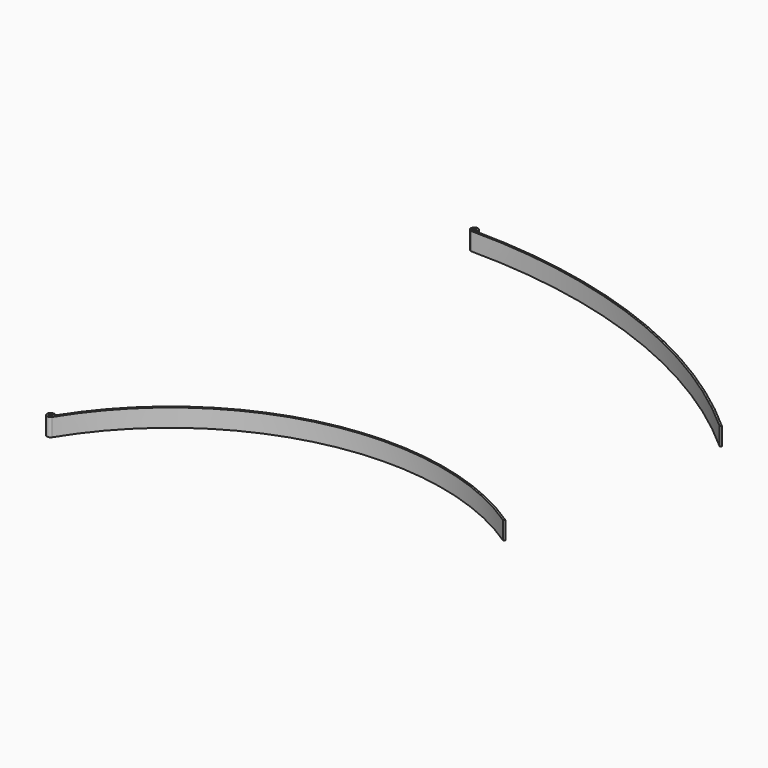
from build123d import *

# Parameters (mm, degrees)
F0_R     = 5
F1_DEPTH = 50
F3_DEPTH = 50


# Not quite as in the source:
# - ends of sketch curves that miss each other by under 0.0002 mm in the source are joined


with BuildPart() as f1:
    # F0 (on Top) → F1 (new body)
    with BuildSketch(Plane.XY):
        with BuildLine():
            Line((0, 1505.0000020167), (0, 1500.0095272064))
            ThreePointArc((0, 1500.0095272064), (4.9828064884, 1501.3393692206), (8.6403438934, 1504.9751993065))
            ThreePointArc((8.6403438934, 1504.9751993065), (4.3201897461, 1504.9938013264), (0, 1505.0000020167))
        make_face()
        with BuildLine():
            ThreePointArc((10, 1510.0095272064), (-7.0710678119, 1517.0805950183), (0, 1500.0095272064))
            Line((0, 1500.0095272064), (0, 1505.0000020167))
            ThreePointArc((0, 1505.0000020167), (4.3201897461, 1504.9938013264), (8.6403438934, 1504.9751993065))
            ThreePointArc((8.6403438934, 1504.9751993065), (9.654103763, 1507.4021759579), (10, 1510.0095272064))
        make_face()
        with Locations((0, 1510.0095272064)):
            Circle(F0_R, mode=Mode.SUBTRACT)
        with BuildLine():
            ThreePointArc((0, 1500), (535.2331346596, 1401.2585384441), (1000, 1118.0339887499))
            Line((1000, 1118.0339887499), (1003.3333346778, 1121.7607702155))
            ThreePointArc((1003.3333346778, 1121.7607702155), (541.0508351311, 1404.3820704759), (8.6403438934, 1504.9751993065))
            ThreePointArc((8.6403438934, 1504.9751993065), (4.9828064884, 1501.3393692206), (0, 1500.0095272064))
            Line((0, 1500.0095272064), (0, 1500))
        make_face()
    extrude(amount=F1_DEPTH)


with BuildPart() as f3:
    # F2 (on Top) → F3 (new body)
    with BuildSketch(Plane.XY):
        with BuildLine():
            ThreePointArc((-165.7523488067, 250.9472365606), (-184.5677200008, 246.5350992369), (-166.051450216, 241.0003994084))
            Line((-166.051450216, 241.0003994084), (-170.3118440891, 243.6174672421))
            ThreePointArc((-170.3118440891, 243.6174672421), (-168.0424024134, 247.2887627444), (-165.7523488067, 250.9472365606))
        make_face()
        with BuildLine():
            ThreePointArc((-169.5722379622, 246.2345350757), (-169.7606909466, 244.8747500496), (-170.3118440891, 243.6174672421))
            ThreePointArc((-170.3118440891, 243.6174672421), (-179.3837849777, 247.5943201019), (-169.5722379622, 246.2345350757))
        make_face(mode=Mode.SUBTRACT)
        with BuildLine():
            Line((-170.3118440891, 243.6174672421), (-166.051454279, 241.0004019042))
            ThreePointArc((-166.051454279, 241.0004019042), (-164.9491439311, 243.5149650235), (-164.5722379622, 246.2345350757))
            ThreePointArc((-164.5722379622, 246.2345350757), (-164.8717510787, 248.6636407183), (-165.7523488067, 250.9472365606))
            ThreePointArc((-165.7523488067, 250.9472365606), (-168.0424024134, 247.2887627444), (-170.3118440891, 243.6174672421))
        make_face()
        with BuildLine():
            ThreePointArc((-166.051454279, 241.0004019042), (321.56850198, 586.9462325741), (908.8224537655, 474.7654159781))
            Line((908.8224537655, 474.7654159781), (911.6111110814, 478.9155175059))
            ThreePointArc((911.6111110814, 478.9155175059), (324.7260159117, 592.7373863711), (-165.7523488067, 250.9472365606))
            ThreePointArc((-165.7523488067, 250.9472365606), (-164.8717510787, 248.6636407183), (-164.5722379622, 246.2345350757))
            ThreePointArc((-164.5722379622, 246.2345350757), (-164.9491439311, 243.5149650235), (-166.051454279, 241.0004019042))
        make_face()
    extrude(amount=F3_DEPTH)


solid = Compound([f1.part, f3.part])
